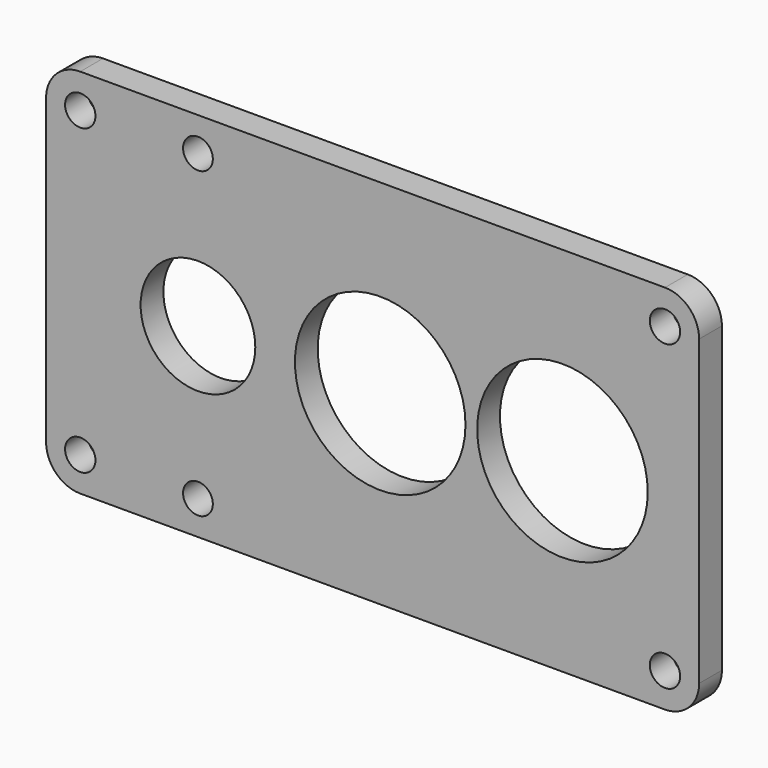
from build123d import *

# Parameters (mm, degrees)
F0_R     = 2.54
F0_R_2   = 2.4892
F0_R_3   = 9.5885
F0_R_4   = 14.2621
F1_DEPTH = 4.7625


# Not quite as in the source:
# - a length typed as a fraction of an inch, garbled in the dataset ("3 / 203.2 mm" for 3/8 in), is restored


with BuildPart() as f1:
    # F0 (on Front) → F1 (new body)
    with BuildSketch(Plane.XZ):
        with BuildLine():
            Line((83.82, -25.3516301214), (83.82, 25.3492))
            ThreePointArc((83.82, 25.3492), (82.1461152545, 29.3903152545), (78.105, 31.0642))
            Line((78.105, 31.0642), (-19.685, 31.0642))
            ThreePointArc((-19.685, 31.0642), (-23.7261152545, 29.3903152545), (-25.4, 25.3492))
            Line((-25.4, 25.3492), (-25.4, -25.3516301214))
            ThreePointArc((-25.4, -25.3516301214), (-23.7915717475, -29.3262110405), (-19.8716383264, -31.0635817261))
            Line((-19.8716383264, -31.0635817261), (-19.4987171118, -31.063593329))
            Line((-19.4987171118, -31.063593329), (78.1048221862, -31.0666301186))
            ThreePointArc((78.1048221862, -31.0666301186), (82.1460523873, -29.392808242), (83.82, -25.3516301214))
        make_face()
        with Locations((-19.685, -25.3516301214)):
            Circle(F0_R, mode=Mode.SUBTRACT)
        with Locations((0, -25.4)):
            Circle(F0_R_2, mode=Mode.SUBTRACT)
        with Locations((78.105, -25.3516301214)):
            Circle(F0_R, mode=Mode.SUBTRACT)
        Circle(F0_R_3, mode=Mode.SUBTRACT)
        with Locations((-19.685, 25.3492)):
            Circle(F0_R, mode=Mode.SUBTRACT)
        with Locations((0, 25.4)):
            Circle(F0_R_2, mode=Mode.SUBTRACT)
        with Locations((30.48, 0)):
            Circle(F0_R_4, mode=Mode.SUBTRACT)
        with Locations((60.96, 0)):
            Circle(F0_R_4, mode=Mode.SUBTRACT)
        with Locations((78.105, 25.3492)):
            Circle(F0_R, mode=Mode.SUBTRACT)
        with BuildLine():
            ThreePointArc((-19.8716383264, -31.0635817261), (-19.6851778138, -31.0666301186), (-19.4987171118, -31.063593329))
            Line((-19.4987171118, -31.063593329), (-19.8716383264, -31.0635817261))
        make_face()
    extrude(amount=F1_DEPTH)


solid = f1.part
